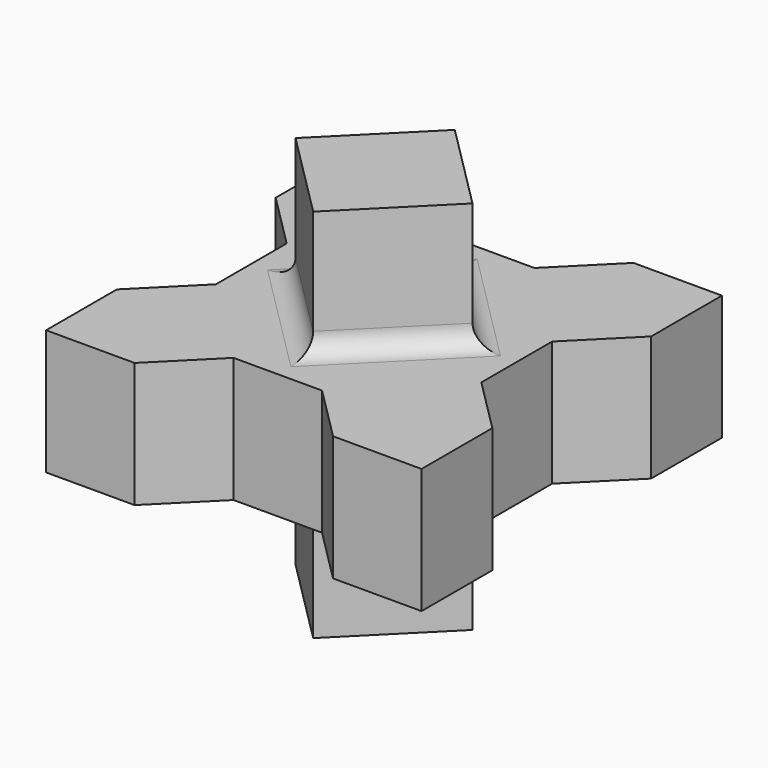
from build123d import *

# Parameters (mm, degrees)
F2_DEPTH = 5
F3_DEPTH = 15
F4_R     = 1.578947


with BuildPart() as f2:
    # F1 (on Top) → F2 (new body, symmetric)
    with BuildSketch(Plane.XY):
        Polygon((-15, -7.928932), (-15, -15), (-7.928932, -15), (-3.535534, -10.606602), (0, -10.606602), (3.535534, -10.606602), (7.928932, -15), (15, -15), (15, -7.928932), (10.606602, -3.535534), (10.606602, 0), (10.606602, 3.535534), (15, 7.928932), (15, 15), (7.928932, 15), (3.535534, 10.606602), (0, 10.606602), (-3.535534, 10.606602), (-7.928932, 15), (-15, 15), (-15, 7.928932), (-10.606602, 3.535534), (-10.606602, 0), (-10.606602, -3.535534), align=None)
        Polygon((3.535534, -3.535534), (0, -7.071068), (-3.535534, -3.535534), (-7.071068, 0), (-3.535534, 3.535534), (0, 7.071068), (3.535534, 3.535534), (7.071068, 0), align=None, mode=Mode.SUBTRACT)
        Polygon((-3.535534, -3.535534), (0, -7.071068), (3.535534, -3.535534), (7.071068, 0), (3.535534, 3.535534), (0, 7.071068), (-3.535534, 3.535534), (-7.071068, 0), align=None)
    extrude(amount=F2_DEPTH, both=True)

    # F1 (on Top) → F3 (join, symmetric)
    with BuildSketch(Plane.XY):
        Polygon((-3.535534, -3.535534), (0, -7.071068), (3.535534, -3.535534), (7.071068, 0), (3.535534, 3.535534), (0, 7.071068), (-3.535534, 3.535534), (-7.071068, 0), align=None)
    extrude(amount=F3_DEPTH, both=True)

    # F4
    f4_edges = [f2.edges().sort_by_distance(p)[0] for p in [
        (-3.535534, -3.535534, 5),
        (3.535534, -3.535534, 5),
        (3.535534, 3.535534, 5),
        (-3.535534, 3.535534, 5),
        (-3.535534, 3.535534, -5),
        (-3.535534, -3.535534, -5),
        (3.535534, -3.535534, -5),
        (3.535534, 3.535534, -5),
    ]]
    fillet(f4_edges, radius=F4_R)


solid = f2.part
